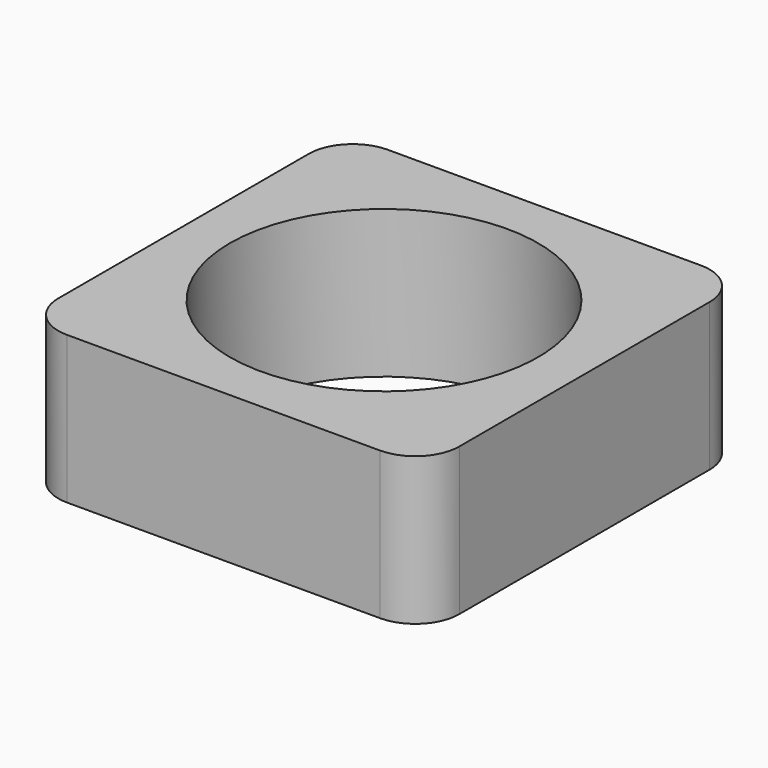
from build123d import *

# Parameters (mm, degrees)
F1_DEPTH = 1.7018
F3_D     = 3.556


# Not quite as in the source:
# - a feature names something its author has since deleted; it is built from what else it names


with BuildPart() as f1:
    # F0 (on Top) → F1 (new body)
    with BuildSketch(Plane.XY):
        with BuildLine():
            Line((2.1907232318, -2.0628636251), (-1.4160767682, -2.0628636251))
            ThreePointArc((-1.4160767682, -2.0628636251), (-1.775287013, -2.2116533802), (-1.9240767682, -2.5708636251))
            Line((-1.9240767682, -2.5708636251), (-1.9240767682, -6.1776636251))
            ThreePointArc((-1.9240767682, -6.1776636251), (-1.775287013, -6.5368738699), (-1.4160767682, -6.6856636251))
            Line((-1.4160767682, -6.6856636251), (2.1907232318, -6.6856636251))
            ThreePointArc((2.1907232318, -6.6856636251), (2.5499334767, -6.5368738699), (2.6987232318, -6.1776636251))
            Line((2.6987232318, -6.1776636251), (2.6987232318, -2.5708636251))
            ThreePointArc((2.6987232318, -2.5708636251), (2.5499334767, -2.2116533802), (2.1907232318, -2.0628636251))
        make_face()
    extrude(amount=F1_DEPTH)

    # F3 (through all)
    with Locations(Plane(origin=(0, 0, 0), x_dir=(1, 0, 0), z_dir=(0, 0, -1))):
        with Locations((0.3873232318, 4.3742636251)):
            Hole(F3_D / 2)


solid = f1.part
